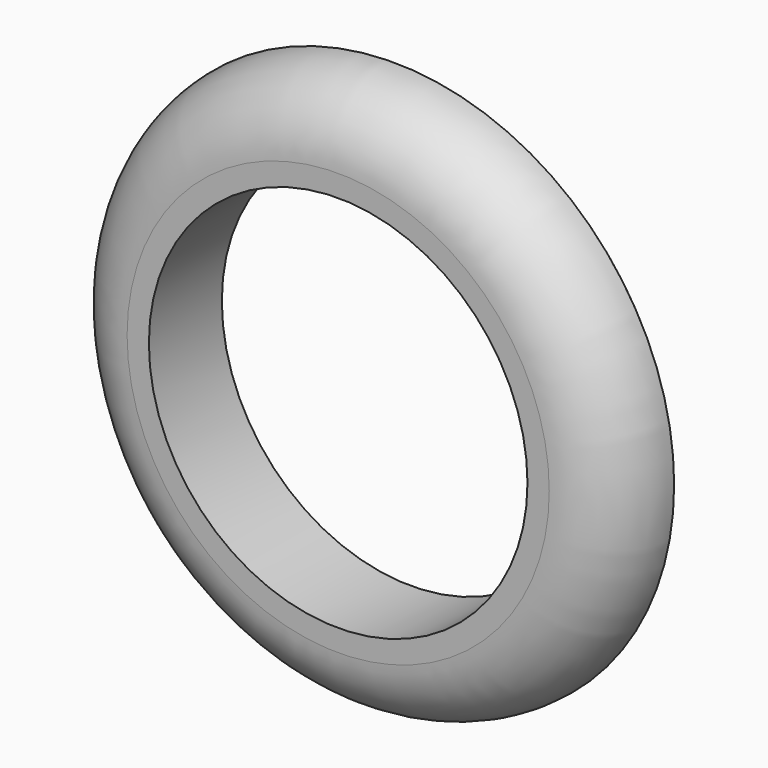
from build123d import *

# Parameters (mm, degrees)
F2_R     = 20.5358515241
F2_R_2   = 13.8603934158
F0_DEPTH = 6.6770780832
F3_R     = 5.08


# Not quite as in the source:
# - a fillet or chamfer that OpenCascade refuses, or shapes differently, is made with other operations: its cross-section is extruded or revolved along the edge and cut away or added


with BuildPart() as f0:
    # F2 (on Front) → F0 (new body)
    with BuildSketch(Plane.XZ):
        Circle(F2_R)
        Circle(F2_R_2, mode=Mode.SUBTRACT)
    extrude(amount=F0_DEPTH)

    # F3
    f3_edges = [f0.edges().sort_by_distance(p)[0] for p in [
        (-20.535852, -6.677078, 0),
    ]]
    fillet(f3_edges, radius=F3_R)

    # F1: fillet of radius 5.08 on 1 edges, made by hand

    # F1_s1 → F1_t2 (revolve, cut)
    with BuildSketch(Plane.XY):
        with BuildLine():
            ThreePointArc((20.5358515241, -1.5970780832), (18.8518854725, -0.4163295926), (16.8377905564, 0))
            Line((16.8377905564, 0), (20.5358515241, 0))
            Line((20.5358515241, 0), (20.5358515241, -1.5970780832))
        make_face()
    revolve(axis=Axis((0, 0, 0), (0, -1, 0)), mode=Mode.SUBTRACT)


solid = f0.part
